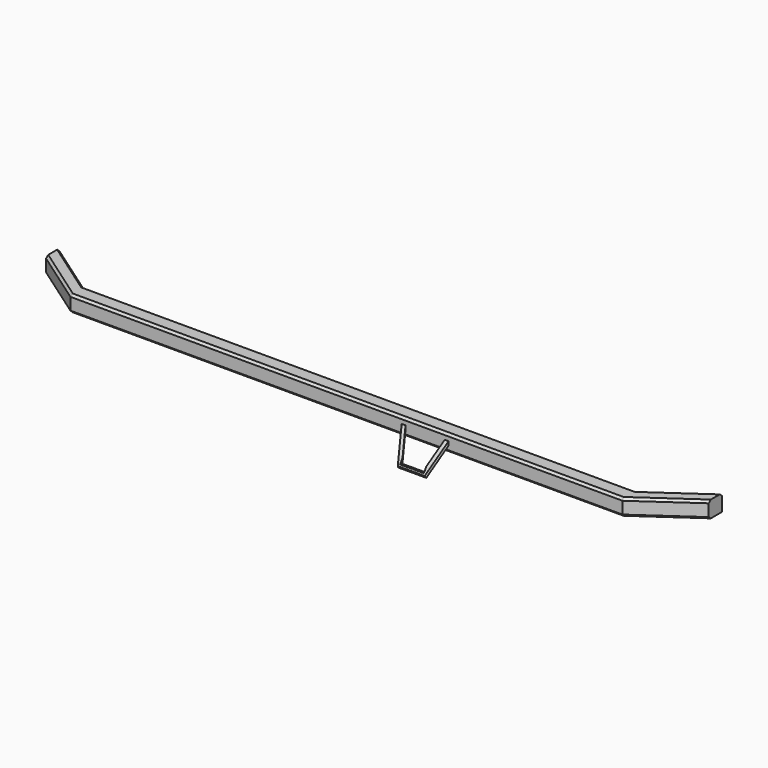
from build123d import *

# Parameters (mm, degrees)
F2_W      = 38.1
F2_H      = 38.1
F6_SIZE   = 5.08
F15_W     = 8.89
F15_H     = 8.89
F20_DEPTH = 76.2
F21_R     = 0.762
F22_DEPTH = 0.762
F22_TAPER = 20


with BuildPart() as f3:
    # F3: sweep along a path in F0
    with BuildLine(Plane.XY) as f3_path:
        Line((635, 0), (762, 88.9))
    # F2 (on plane+point) → F3 (sweep)
    with BuildSketch(Plane.YZ.offset(635)):
        Rectangle(F2_W, F2_H)
    sweep(path=f3_path.line)

    # F4: sweep along a path in F0
    with BuildLine(Plane.XY) as f4_path:
        Line((0, 0), (635, 0))
    # F2 (on plane+point) → F4 (sweep)
    with BuildSketch(Plane.YZ.offset(635)):
        Rectangle(F2_W, F2_H)
    sweep(path=f4_path.line)

    # F5: F3 across plane


with BuildPart() as f3_1:
    add(f3.part)
    add(f3.part.mirror(Plane.YZ))

    # F6
    f6_edges = [f3_1.edges().sort_by_distance(p)[0] for p in [
        (0, -19.05, 19.05),
        (-698.5, 25.4, 19.05),
        (-698.5, 63.5, 19.05),
        (0, 19.05, 19.05),
        (-698.5, 25.4, -19.05),
        (0, -19.05, -19.05),
        (698.5, 25.4, 19.05),
        (698.5, 63.5, 19.05),
        (698.5, 25.4, -19.05),
    ]]
    chamfer(f6_edges, length=F6_SIZE)

    # F17: sweep along a path in F17_path
    with BuildLine(Plane(origin=(230.4893882996, -19.05, 0), x_dir=(0, -0.5448669245, -0.8385225308), z_dir=(0, 0.8385225308, -0.5448669245))) as f17_path:
        Line((0, 0), (66.6308678854, 20.9606761542))
        Line((66.6308678854, 20.9606761542), (66.6308678854, 78.1106761542))
        Line((66.6308678854, 78.1106761542), (0, 99.0713523085))
        Line((0, 99.0713523085), (-9.6917626015, 102.1201779309))
    # F15 (on face) → F17 (sweep)
    with BuildSketch(Plane.XZ.offset(19.05)):
        with Locations((230.4893882996, 0)):
            Rectangle(F15_W, F15_H)
    sweep(path=f17_path.line, transition=Transition.RIGHT)

    # F19 (on face) → F20 (cut)
    with BuildSketch(Plane.XZ.offset(59.0866984684)):
        Polygon((180.9537121453, -41.0576526403), (153.6487121453, -41.0576526403), (153.6487121453, -53.7576526403), (180.9537121453, -53.7576526403), (208.2587121453, -53.7576526403), (208.2587121453, -41.0576526403), align=None)
    extrude(amount=-F20_DEPTH, mode=Mode.SUBTRACT)


with BuildPart() as f22:
    # F21 (on face) → F22 (new body)
    with BuildSketch(Plane.XY.offset(-53.7576526403)):
        with Locations((159.9987121453, -55.7267355194)):
            Circle(F21_R)
    extrude(amount=F22_DEPTH, taper=F22_TAPER)


with BuildPart() as f22b:
    # F21 (on face) → F22, piece 2 (new body)
    with BuildSketch(Plane.XY.offset(-53.7576526403)):
        with Locations((170.4762121453, -55.7267355194)):
            Circle(F21_R)
    extrude(amount=F22_DEPTH, taper=F22_TAPER)


with BuildPart() as f22c:
    # F21 (on face) → F22, piece 3 (new body)
    with BuildSketch(Plane.XY.offset(-53.7576526403)):
        with Locations((180.9537121453, -55.7267355194)):
            Circle(F21_R)
    extrude(amount=F22_DEPTH, taper=F22_TAPER)


with BuildPart() as f22d:
    # F21 (on face) → F22, piece 4 (new body)
    with BuildSketch(Plane.XY.offset(-53.7576526403)):
        with Locations((191.4312121453, -55.7267355194)):
            Circle(F21_R)
    extrude(amount=F22_DEPTH, taper=F22_TAPER)


with BuildPart() as f22e:
    # F21 (on face) → F22, piece 5 (new body)
    with BuildSketch(Plane.XY.offset(-53.7576526403)):
        with Locations((201.9087121453, -55.7267355194)):
            Circle(F21_R)
    extrude(amount=F22_DEPTH, taper=F22_TAPER)


with BuildPart() as f22f:
    # F21 (on face) → F22, piece 6 (new body)
    with BuildSketch(Plane.XY.offset(-53.7576526403)):
        with Locations((159.9987121453, -53.2883355194)):
            Circle(F21_R)
    extrude(amount=F22_DEPTH, taper=F22_TAPER)


with BuildPart() as f22g:
    # F21 (on face) → F22, piece 7 (new body)
    with BuildSketch(Plane.XY.offset(-53.7576526403)):
        with Locations((170.4762119939, -53.2883355194)):
            Circle(F21_R)
    extrude(amount=F22_DEPTH, taper=F22_TAPER)


with BuildPart() as f22h:
    # F21 (on face) → F22, piece 8 (new body)
    with BuildSketch(Plane.XY.offset(-53.7576526403)):
        with Locations((180.9537118425, -53.2883355194)):
            Circle(F21_R)
    extrude(amount=F22_DEPTH, taper=F22_TAPER)


with BuildPart() as f22i:
    # F21 (on face) → F22, piece 9 (new body)
    with BuildSketch(Plane.XY.offset(-53.7576526403)):
        with Locations((191.4312116911, -53.2883355194)):
            Circle(F21_R)
    extrude(amount=F22_DEPTH, taper=F22_TAPER)


with BuildPart() as f22j:
    # F21 (on face) → F22, piece 10 (new body)
    with BuildSketch(Plane.XY.offset(-53.7576526403)):
        with Locations((201.9087115398, -53.2883355194)):
            Circle(F21_R)
    extrude(amount=F22_DEPTH, taper=F22_TAPER)


solid = Compound([f3_1.part, f22.part, f22b.part, f22c.part, f22d.part, f22e.part, f22f.part, f22g.part, f22h.part, f22i.part, f22j.part])
